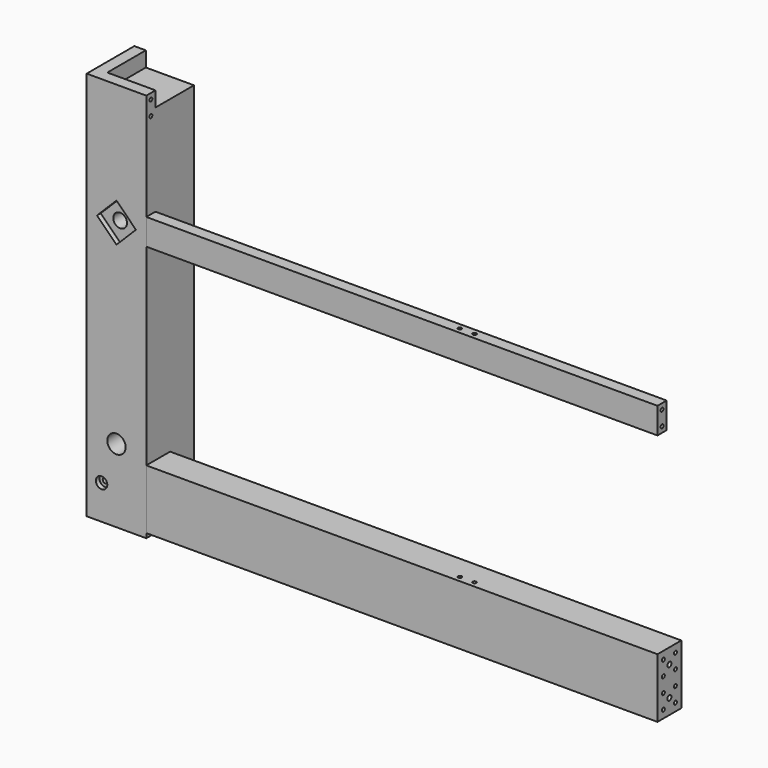
from build123d import *

# Parameters (mm, degrees)
F0_W      = 130
F0_H      = 130
F1_DEPTH  = 850
F2_R      = 15
F2_R_2    = 20
F2_R_3    = 5.5
F3_DEPTH  = 130.001
F4_R      = 5.5
F5_DEPTH  = 140
F6_W      = 105
F6_H      = 105
F7_DEPTH  = 33
F8_R      = 4
F9_DEPTH  = 20
F10_R     = 4
F11_DEPTH = 20
F12_R     = 12.5
F13_DEPTH = 10
F14_R     = 12.5
F15_DEPTH = 10
F16_W     = 65
F16_H     = 130
F17_DEPTH = 1115
F18_R     = 4
F18_R_2   = 5.5
F19_DEPTH = 40
F20_R     = 4
F20_R_2   = 5.5
F21_DEPTH = 40
F22_R     = 4
F23_DEPTH = 20
F24_W     = 25
F24_H     = 57
F25_DEPTH = 1115
F26_R     = 4
F27_DEPTH = 20
F28_R     = 4
F29_DEPTH = 20
F30_R     = 4
F31_DEPTH = 617.001


with BuildPart() as f1:
    # F0 (on Top) → F1 (new body)
    with BuildSketch(Plane.XY):
        with Locations((65, -65)):
            Rectangle(F0_W, F0_H)
    extrude(amount=F1_DEPTH)

    # F2 (on face) → F3 (cut, through all)
    with BuildSketch(Plane.XZ.offset(130)):
        with Locations((65, 585)):
            Circle(F2_R)
        with Locations((65, 160)):
            Circle(F2_R_2)
        with Locations((32.5, 75)):
            Circle(F2_R_3)
    extrude(amount=-F3_DEPTH, mode=Mode.SUBTRACT)

    # F4 (on face) → F5 (cut)
    with BuildSketch(Plane.YZ.offset(130)):
        with Locations((-97.5, 107)):
            Circle(F4_R)
        with Locations((-97.5, 43)):
            Circle(F4_R)
    extrude(amount=-F5_DEPTH, mode=Mode.SUBTRACT)

    # F6 (on face) → F7 (cut)
    with BuildSketch(Plane.XY.offset(850)):
        with Locations((77.5, -52.5)):
            Rectangle(F6_W, F6_H)
    extrude(amount=-F7_DEPTH, mode=Mode.SUBTRACT)

    # F8 (on face) → F9 (cut)
    with BuildSketch(Plane.YZ.offset(130)):
        with Locations((-114, 123)):
            Circle(F8_R)
        with Locations((-81, 123)):
            Circle(F8_R)
        with Locations((-114, 91)):
            Circle(F8_R)
        with Locations((-81, 91)):
            Circle(F8_R)
        with Locations((-114, 59)):
            Circle(F8_R)
        with Locations((-81, 59)):
            Circle(F8_R)
        with Locations((-114, 27)):
            Circle(F8_R)
        with Locations((-81, 27)):
            Circle(F8_R)
        with Locations((-117.5, 837.5)):
            Circle(F8_R)
        with Locations((-117.5, 805.5)):
            Circle(F8_R)
        with Locations((-117.5, 604.5)):
            Circle(F8_R)
        with Locations((-117.5, 572.5)):
            Circle(F8_R)
    extrude(amount=-F9_DEPTH, mode=Mode.SUBTRACT)

    # F10 (on face) → F11 (cut)
    with BuildSketch(Plane(origin=(0, 0, 0), x_dir=(-1, 0, 0), z_dir=(0, 1, 0))):
        with Locations((-16.25, 123)):
            Circle(F10_R)
        with Locations((-16.25, 91)):
            Circle(F10_R)
        with Locations((-48.75, 123)):
            Circle(F10_R)
        with Locations((-48.75, 91)):
            Circle(F10_R)
        with Locations((-48.75, 27)):
            Circle(F10_R)
        with Locations((-16.25, 27)):
            Circle(F10_R)
        with Locations((-16.25, 59)):
            Circle(F10_R)
        with Locations((-48.75, 59)):
            Circle(F10_R)
        with Locations((-12.5, 837.5)):
            Circle(F10_R)
        with Locations((-12.5, 805.5)):
            Circle(F10_R)
        with Locations((-14.2287150467, 605.5064407267)):
            Circle(F10_R)
        with Locations((-14.2287150467, 573.5064407267)):
            Circle(F10_R)
    extrude(amount=-F11_DEPTH, mode=Mode.SUBTRACT)

    # F12 (on face) → F13 (cut)
    with BuildSketch(Plane.XZ.offset(130)):
        Polygon((22.5735931288, 585), (65, 542.5735931288), (107.4264068712, 585), (65, 627.4264068712), align=None)
        with Locations((32.5, 75)):
            Circle(F12_R)
    extrude(amount=-F13_DEPTH, mode=Mode.SUBTRACT)

    # F14 (on face) → F15 (cut)
    with BuildSketch(Plane(origin=(0, 0, 0), x_dir=(0, -1, 0), z_dir=(-1, 0, 0))):
        with Locations((97.5, 107)):
            Circle(F14_R)
        with Locations((97.5, 43)):
            Circle(F14_R)
    extrude(amount=-F15_DEPTH, mode=Mode.SUBTRACT)


with BuildPart() as f17:
    # F16 (on face) → F17 (new body)
    with BuildSketch(Plane.YZ.offset(130)):
        with Locations((-97.5, 75)):
            Rectangle(F16_W, F16_H)
    extrude(amount=F17_DEPTH)

    # F18 (on face) → F19 (cut)
    with BuildSketch(Plane.YZ.offset(1245)):
        with Locations((-114, 123)):
            Circle(F18_R)
        with Locations((-81, 123)):
            Circle(F18_R)
        with Locations((-81, 91)):
            Circle(F18_R)
        with Locations((-114, 91)):
            Circle(F18_R)
        with Locations((-114, 59)):
            Circle(F18_R)
        with Locations((-81, 59)):
            Circle(F18_R)
        with Locations((-81, 27)):
            Circle(F18_R)
        with Locations((-114, 27)):
            Circle(F18_R)
        with Locations((-97.5, 43)):
            Circle(F18_R_2)
        with Locations((-97.5, 107)):
            Circle(F18_R_2)
    extrude(amount=-F19_DEPTH, mode=Mode.SUBTRACT)

    # F20 (on face) → F21 (cut)
    with BuildSketch(Plane(origin=(130, 0, 0), x_dir=(0, -1, 0), z_dir=(-1, 0, 0))):
        with Locations((81, 123)):
            Circle(F20_R)
        with Locations((97.5, 107)):
            Circle(F20_R_2)
        with Locations((114, 123)):
            Circle(F20_R)
        with Locations((114, 91)):
            Circle(F20_R)
        with Locations((114, 59)):
            Circle(F20_R)
        with Locations((114, 27)):
            Circle(F20_R)
        with Locations((97.5, 43)):
            Circle(F20_R_2)
        with Locations((81, 27)):
            Circle(F20_R)
        with Locations((81, 59)):
            Circle(F20_R)
        with Locations((81, 91)):
            Circle(F20_R)
    extrude(amount=-F21_DEPTH, mode=Mode.SUBTRACT)

    # F22 (on face) → F23 (cut)
    with BuildSketch(Plane.XY.offset(140)):
        with Locations((804, -117.5)):
            Circle(F22_R)
        with Locations((836, -117.5)):
            Circle(F22_R)
    extrude(amount=-F23_DEPTH, mode=Mode.SUBTRACT)


with BuildPart() as f25:
    # F24 (on face) → F25 (new body)
    with BuildSketch(Plane.YZ.offset(130)):
        with Locations((-117.5, 588.5)):
            Rectangle(F24_W, F24_H)
    extrude(amount=F25_DEPTH)

    # F26 (on face) → F27 (cut)
    with BuildSketch(Plane.YZ.offset(1245)):
        with Locations((-117.5, 604.5)):
            Circle(F26_R)
        with Locations((-117.5, 572.5)):
            Circle(F26_R)
    extrude(amount=-F27_DEPTH, mode=Mode.SUBTRACT)

    # F28 (on face) → F29 (cut)
    with BuildSketch(Plane(origin=(130, 0, 0), x_dir=(0, -1, 0), z_dir=(-1, 0, 0))):
        with Locations((117.5, 604.5)):
            Circle(F28_R)
        with Locations((117.5, 572.5)):
            Circle(F28_R)
    extrude(amount=-F29_DEPTH, mode=Mode.SUBTRACT)

    # F30 (on face) → F31 (cut, through all)
    with BuildSketch(Plane.XY.offset(617)):
        with Locations((804, -117.5)):
            Circle(F30_R)
        with Locations((836, -117.5)):
            Circle(F30_R)
    extrude(amount=-F31_DEPTH, mode=Mode.SUBTRACT)


solid = Compound([f1.part, f17.part, f25.part])
